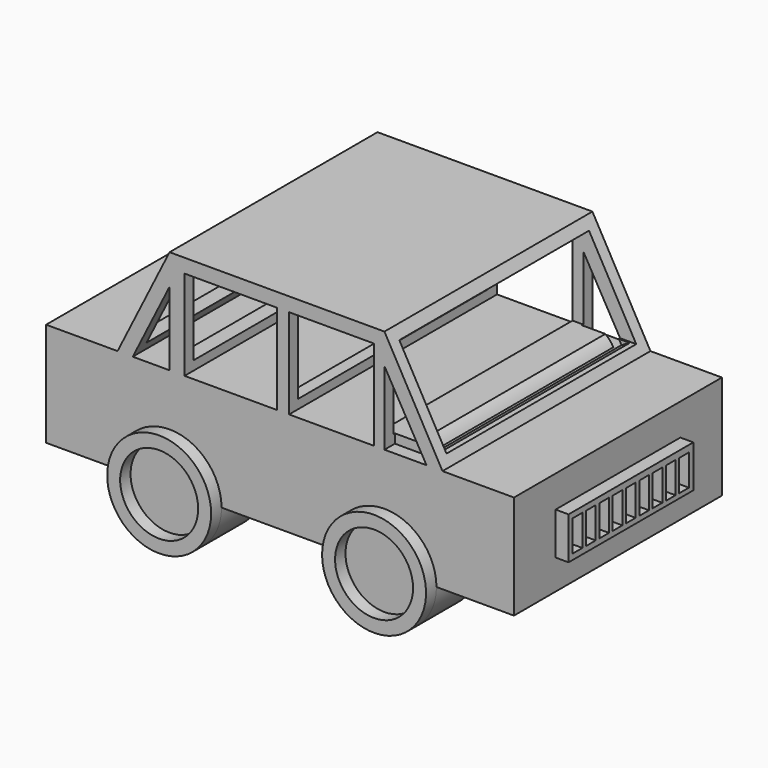
from build123d import *

# Parameters (mm, degrees)
F0_W       = 228.6
F0_H       = 50.8
F1_DEPTH   = 63.5
F2_R       = 25.4
F3_DEPTH   = 25.4
F5_W       = 133.35
F5_H       = 127
F6_DEPTH   = 50.8
F8_DEPTH   = 127.001
F9_W       = 114.3
F9_H       = 45.4757122113
F10_DEPTH  = 25.4
F11_DEPTH  = 25.4
F13_DEPTH  = 127.001
F14_W      = 45.1612845063
F14_H      = 43.987744288
F14_W_2    = 41.4102021605
F15_DEPTH  = 127.001
F15_FACE_W = 114.3
F15_FACE_H = 14.0218776853
F18_W      = 115.8576831222
F18_H      = 41.3168929517
F19_DEPTH  = 191.9764496515
F20_W      = 76.2
F20_H      = 20.6366241442
F20_W_2    = 5.92666582
F20_H_2    = 15.1961888187
F21_DEPTH  = 6.35
F22_R      = 19.05
F23_DEPTH  = 6.35
F24_R      = 19.05
F25_DEPTH  = 6.35


with BuildPart() as f1:
    # F0 (on Front) → F1 (new body, symmetric)
    with BuildSketch(Plane.XZ):
        with Locations((1.4754496515, 2.5203571515)):
            Rectangle(F0_W, F0_H)
    extrude(amount=F1_DEPTH, both=True)

    # F2 (on face) → F3 (join)
    with BuildSketch(Plane.XZ.offset(63.5)):
        with BuildLine():
            ThreePointArc((-77.8995503485, -22.8796428485), (-52.4995503485, -48.2796428485), (-27.0995503485, -22.8796428485))
            ThreePointArc((-27.0995503485, -22.8796428485), (-52.4995503485, 2.5203571515), (-77.8995503485, -22.8796428485))
        make_face()
        with Locations((52.4995503485, -22.8796428485)):
            Circle(F2_R)
    extrude(amount=-F3_DEPTH)

    # F4: F1 across plane


with BuildPart() as f1_1:
    add(f1.part)
    add(f1.part.mirror(Plane.XZ))

    # F5 (on face) → F6 (join)
    with BuildSketch(Plane.XY.offset(27.9203571515)):
        with Locations((14.1754496515, 0)):
            Rectangle(F5_W, F5_H)
    extrude(amount=F6_DEPTH)

    # F7 (on face) → F8 (cut, through all)
    with BuildSketch(Plane.XZ.offset(63.5)):
        Polygon((80.8504496515, 78.7203571515), (52.4995503485, 78.7203571515), (80.8504496515, 27.9203571515), align=None)
    extrude(amount=-F8_DEPTH, mode=Mode.SUBTRACT)

    # F9 (on face) → F10 (cut)
    with BuildSketch(Plane(origin=(73.5304715342, 0, 41.0365156332), x_dir=(0, 1, 0), z_dir=(0.8732166409, 0, 0.4873322255))):
        with Locations((0, 14.0673470279)):
            Rectangle(F9_W, F9_H)
    extrude(amount=-F10_DEPTH, mode=Mode.SUBTRACT)

    # F11 (add): a face of the model
    f11_faces = [f1_1.faces().sort_by_distance(p)[0] for p in [
        (-52.4995503485, 0, 53.3203571515),
    ]]
    extrude(f11_faces, amount=F11_DEPTH)

    # F12 (on face) → F13 (cut, through all)
    with BuildSketch(Plane.XZ.offset(63.5)):
        Polygon((-77.8995503485, 78.7203571515), (-77.8995503485, 27.9203571515), (-52.4995503485, 78.7203571515), align=None)
    extrude(amount=-F13_DEPTH, mode=Mode.SUBTRACT)

    # F14 (on face) → F15 (cut, through all)
    with BuildSketch(Plane.XZ.offset(63.5)):
        Polygon((-52.4995503485, 27.9203571515), (-52.4995503485, 63.8672858477), (-70.4730146966, 27.9203571515), align=None)
        with Locations((-22.5806422532, 49.9142292955)):
            Rectangle(F14_W, F14_H)
        with Locations((26.6029974446, 49.9142292955)):
            Rectangle(F14_W_2, F14_H)
        Polygon((73.0387046933, 27.9203571515), (52.4995503485, 63.8672858477), (52.4995503485, 27.9203571515), align=None)
    extrude(amount=-F15_DEPTH, mode=Mode.SUBTRACT)

    # F15_face (on face) → F16 (revolve)
    with BuildSketch(Plane(origin=(61.698255806, 0, 24.5037007223), x_dir=(0, -1, 0), z_dir=(-0.4873322255, 0, 0.8732166409))):
        Rectangle(F15_FACE_W, F15_FACE_H)
    revolve(axis=Axis((55.5761873402, 0, 21.0870442932), (0, -1, 0)))

    # F18 (on offset) → F19 (cut, through all)
    with BuildSketch(Plane.YZ.offset(-76.2)):
        with Locations((7.4506e-06, 53.0304405838)):
            Rectangle(F18_W, F18_H)
    extrude(amount=F19_DEPTH, mode=Mode.SUBTRACT)

    # F20 (on face) → F21 (join)
    with BuildSketch(Plane.YZ.offset(115.7754496515)):
        with Locations((0, 2.0944098942)):
            Rectangle(F20_W, F20_H)
        with Locations((-32.59666709, 2.1173956338)):
            Rectangle(F20_W_2, F20_H_2, mode=Mode.SUBTRACT)
        with Locations((-24.4689150477, 2.0539075275)):
            Rectangle(F20_W_2, F20_H_2, mode=Mode.SUBTRACT)
        with Locations((-16.3411630055, 1.9904194212)):
            Rectangle(F20_W_2, F20_H_2, mode=Mode.SUBTRACT)
        with Locations((-8.2134109632, 1.9269313149)):
            Rectangle(F20_W_2, F20_H_2, mode=Mode.SUBTRACT)
        with Locations((-0.085658921, 1.8634432086)):
            Rectangle(F20_W_2, F20_H_2, mode=Mode.SUBTRACT)
        with Locations((8.0420931213, 1.7999551023)):
            Rectangle(F20_W_2, F20_H_2, mode=Mode.SUBTRACT)
        with Locations((16.1698451635, 1.736466996)):
            Rectangle(F20_W_2, F20_H_2, mode=Mode.SUBTRACT)
        with Locations((24.2975972058, 1.6729788898)):
            Rectangle(F20_W_2, F20_H_2, mode=Mode.SUBTRACT)
        with Locations((32.425349248, 1.6094907835)):
            Rectangle(F20_W_2, F20_H_2, mode=Mode.SUBTRACT)
    extrude(amount=F21_DEPTH)

    # F22 (on face) → F23 (join)
    with BuildSketch(Plane(origin=(0, 63.5, 0), x_dir=(-1, 0, 0), z_dir=(0, 1, 0))):
        with BuildLine():
            ThreePointArc((-77.8995503485, -22.8796428485), (-52.4995503485, -48.2796428485), (-27.0995503485, -22.8796428485))
            ThreePointArc((-27.0995503485, -22.8796428485), (-52.4995503485, 2.5203571515), (-77.8995503485, -22.8796428485))
        make_face()
        with Locations((-52.4995503485, -22.8796428485)):
            Circle(F22_R, mode=Mode.SUBTRACT)
        with BuildLine():
            ThreePointArc((77.8995503485, -22.8796428485), (52.4995503485, 2.5203571515), (27.0995503485, -22.8796428485))
            ThreePointArc((27.0995503485, -22.8796428485), (52.4995503485, -48.2796428485), (77.8995503485, -22.8796428485))
        make_face()
        with Locations((52.4995503485, -22.8796428485)):
            Circle(F22_R, mode=Mode.SUBTRACT)
    extrude(amount=F23_DEPTH)

    # F24 (on face) → F25 (join)
    with BuildSketch(Plane.XZ.offset(63.5)):
        with BuildLine():
            ThreePointArc((-77.8995503485, -22.8796428485), (-52.4995503485, -48.2796428485), (-27.0995503485, -22.8796428485))
            ThreePointArc((-27.0995503485, -22.8796428485), (-52.4995503485, 2.5203571515), (-77.8995503485, -22.8796428485))
        make_face()
        with Locations((-52.4995503485, -22.8796428485)):
            Circle(F24_R, mode=Mode.SUBTRACT)
        with BuildLine():
            ThreePointArc((77.8995503485, -22.8796428485), (52.4995503485, 2.5203571515), (27.0995503485, -22.8796428485))
            ThreePointArc((27.0995503485, -22.8796428485), (52.4995503485, -48.2796428485), (77.8995503485, -22.8796428485))
        make_face()
        with Locations((52.4995503485, -22.8796428485)):
            Circle(F24_R, mode=Mode.SUBTRACT)
    extrude(amount=F25_DEPTH)


solid = f1_1.part
